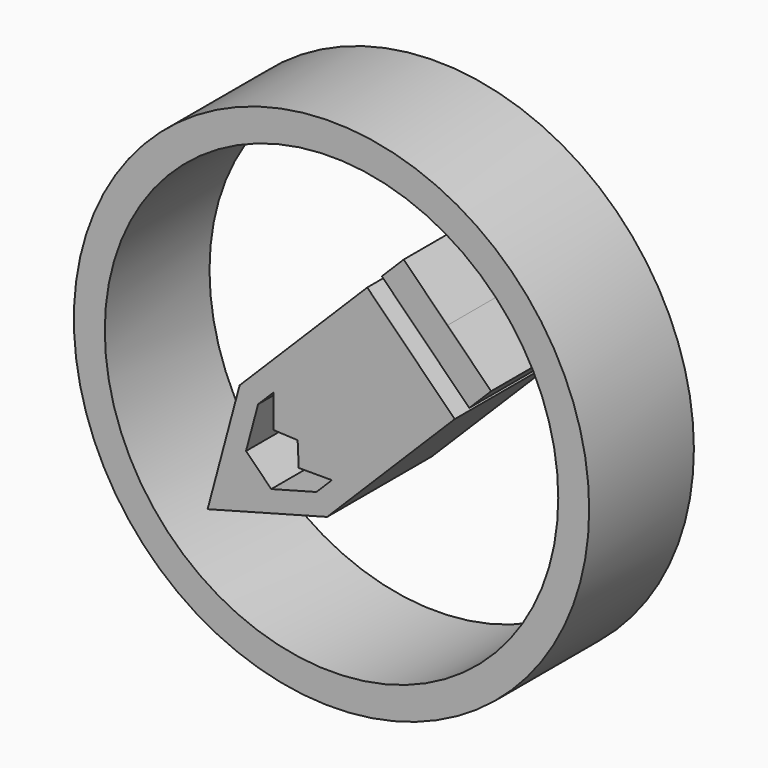
from build123d import *

# Parameters (mm, degrees)
F0_R     = 50
F0_R_2   = 44
F1_DEPTH = 25.4
F2_DEPTH = 25.4


# Not quite as in the source:
# - a feature names something its author has since deleted; it is built from what else it names


with BuildPart() as f1:
    # F0 (on Front) → F1 (new body)
    with BuildSketch(Plane.XZ):
        Circle(F0_R)
        Circle(F0_R_2, mode=Mode.SUBTRACT)
    extrude(amount=F1_DEPTH)


with BuildPart() as f2:
    # F0 (on Front) → F2 (new body)
    with BuildSketch(Plane.XZ):
        Polygon((-24.0416305603, -24.0416305603), (-18.3847763109, -18.3847763109), (-16.5916253665, -11.6926458809), (-19.8576116902, -8.4266595572), align=None)
        Polygon((-18.3847763109, -18.3847763109), (-14.1421356237, -14.1421356237), (-16.5916253665, -11.6926458809), align=None)
        Polygon((-11.2475056175, 0.0662028815), (9.7607779651, 21.0744864641), (6.9323508404, 23.9029135888), (-17.8299734779, -0.8594107294), (-19.8576116902, -8.4266595572), (-16.5916253665, -11.6926458809), (-14.2436715892, -2.9299630902), align=None)
        Polygon((-6.5731576178, -6.5731576178), (0, 0), (15.4176322146, 15.4176322146), (9.7607779651, 21.0744864641), (-11.2475056175, 0.0662028815), (-11.2475056175, -6.3611790538), align=None)
    extrude(amount=F2_DEPTH)

    # F3: F2 across face


with BuildPart() as f2b:
    # F0 (on Front) → F2, piece 2 (new body)
    with BuildSketch(Plane.XZ):
        Polygon((14.0034186522, 30.9739814007), (9.7607779651, 26.7313407136), (18.2460593393, 18.2460593393), (22.4887000265, 22.4887000265), align=None)
    extrude(amount=F2_DEPTH)

    # F4: F2b across face


with BuildPart() as f2_1:
    add(f2.part)
    add(f2.part.mirror(Plane(origin=(4.4222372984, -12.7, 4.4222372984), x_dir=(0, 1, 0), z_dir=(0.7071067812, 0, -0.7071067812))))


with BuildPart() as f2b_1:
    add(f2b.part)
    add(f2b.part.mirror(Plane(origin=(20.3673796829, -12.7, 20.3673796829), x_dir=(0, 1, 0), z_dir=(0.7071067812, 0, -0.7071067812))))


solid = Compound([f1.part, f2_1.part, f2b_1.part])
